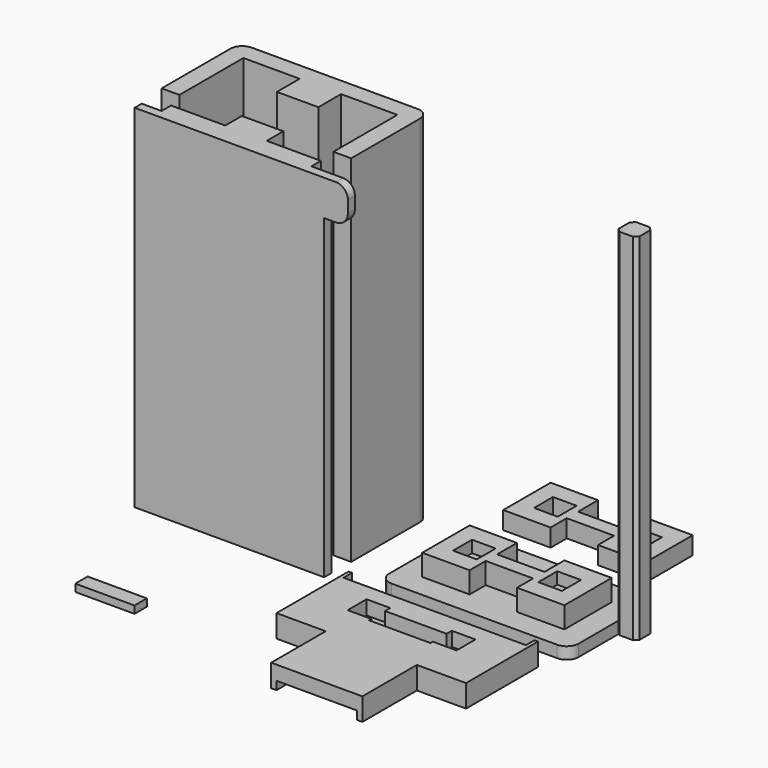
from build123d import *

# Parameters (mm, degrees)
F0_W      = 30.48
F0_H      = 12.7
F1_DEPTH  = 4.572
F2_W      = 5.08
F2_H      = 5.08
F3_DEPTH  = 2.54
F2_H_2    = 1.524
F2_H_3    = 3.81
F2_H_4    = 4.318
F4_DEPTH  = 7.62
F6_DEPTH  = 2.54
F8_DEPTH  = 76.2
F9_W      = 5.08
F9_H      = 5.08
F10_DEPTH = 3.81
F11_W     = 8.89
F11_H     = 6.096
F12_DEPTH = 76.2
F14_DEPTH = 4.826
F15_DEPTH = 1.778
F16_W     = 17.272
F16_H     = 1.778
F17_DEPTH = 3.81
F18_W     = 12.7
F18_H     = 3.302
F19_DEPTH = 1.5875
F20_W     = 8.89
F20_H     = 4.445
F21_DEPTH = 75.438
F22_W     = 1.905
F22_H     = 7.62
F23_DEPTH = 5.08
F24_R     = 2.54
F25_R     = 2.54


# Not quite as in the source:
# - a feature names something its author has since deleted; it is built from what else it names


with BuildPart() as f1:
    # F0 (on Top) → F1 (new body)
    with BuildSketch(Plane.XY):
        Rectangle(F0_W, F0_H)
    extrude(amount=F1_DEPTH)

    # F2 (on face) → F3 (cut)
    with BuildSketch(Plane.XY.offset(4.572)):
        with Locations((-9.144, 0)):
            Rectangle(F2_W, F2_H)
        with Locations((9.144, 0)):
            Rectangle(F2_W, F2_H)
    extrude(amount=-F3_DEPTH, mode=Mode.SUBTRACT)

    # F2 (on face) → F4 (cut)
    with BuildSketch(Plane.XY.offset(4.572)):
        with Locations((-2.54, 1.778)):
            Rectangle(F2_W, F2_H_2)
        with Locations((-2.54, 4.445)):
            Rectangle(F2_W, F2_H_3)
        Polygon((5.08, 6.35), (0, 6.35), (0, 2.54), (0, 1.016), (5.08, 1.016), align=None)
        with Locations((2.54, -4.191)):
            Rectangle(F2_W, F2_H_4)
        with Locations((-2.54, -4.191)):
            Rectangle(F2_W, F2_H_4)
    extrude(amount=-F4_DEPTH, mode=Mode.SUBTRACT)

    # F5 (on face) → F6 (join)
    with BuildSketch(Plane(origin=(0, 0, 0), x_dir=(1, 0, 0), z_dir=(0, 0, -1))):
        with BuildLine():
            Line((-20.32, -6.8208193406), (-20.32, -8.89))
            ThreePointArc((-20.32, -8.89), (-19.5760512242, -10.6860512242), (-17.78, -11.43))
            Line((-17.78, -11.43), (-17.2756779939, -11.43))
            Line((-17.2756779939, -11.43), (17.78, -11.43))
            ThreePointArc((17.78, -11.43), (19.5760512242, -10.6860512242), (20.32, -8.89))
            Line((20.32, -8.89), (20.32, 0))
            Line((20.32, 0), (20.32, 8.89))
            ThreePointArc((20.32, 8.89), (19.5760512242, 10.6860512242), (17.78, 11.43))
            Line((17.78, 11.43), (0, 11.43))
            Line((0, 11.43), (-17.78, 11.43))
            ThreePointArc((-17.78, 11.43), (-19.5760512242, 10.6860512242), (-20.32, 8.89))
            Line((-20.32, 8.89), (-20.32, -6.8208193406))
        make_face()
        Polygon((5.08, 6.35), (15.24, 6.35), (15.24, -6.35), (5.08, -6.35), (5.08, -1.016), (-5.08, -1.016), (-5.08, -6.35), (-15.24, -6.35), (-15.24, 6.35), (-5.08, 6.35), (-5.08, 2.032), (5.08, 2.032), align=None, mode=Mode.SUBTRACT)
        Polygon((15.24, -6.35), (15.24, 6.35), (5.08, 6.35), (5.08, 2.032), (-5.08, 2.032), (-5.08, 6.35), (-15.24, 6.35), (-15.24, -6.35), (-5.08, -6.35), (-5.08, -1.016), (5.08, -1.016), (5.08, -6.35), align=None)
    extrude(amount=F6_DEPTH)


with BuildPart() as f8:
    # F7 (on Top) → F8 (new body)
    with BuildSketch(Plane.XY):
        Polygon((27.4387739635, 1.4605), (26.6767739635, 2.2225), (23.7557739635, 2.2225), (22.9937739635, 1.4605), (22.9937739635, -1.4605), (23.7557739635, -2.2225), (25.2162739635, -2.2225), (26.6767739635, -2.2225), (27.4387739635, -1.4605), (27.4387739635, 0), align=None)
    extrude(amount=F8_DEPTH)


with BuildPart() as f10:
    # F9 (on Top) → F10 (new body)
    with BuildSketch(Plane.XY):
        Polygon((15.24, 15.3667641968), (15.24, 28.0667641968), (5.08, 28.0667641968), (5.08, 22.7327641968), (0, 22.7327641968), (-5.08, 22.7327641968), (-5.08, 24.2567641968), (-5.08, 28.0667641968), (-15.24, 28.0667641968), (-15.24, 15.3667641968), (-5.08, 15.3667641968), (-5.08, 19.6847641968), (0, 19.6847641968), (5.08, 19.6847641968), (5.08, 15.3667641968), align=None)
        with Locations((-9.144, 21.7167641968)):
            Rectangle(F9_W, F9_H, mode=Mode.SUBTRACT)
        with Locations((9.144, 21.7167641968)):
            Rectangle(F9_W, F9_H, mode=Mode.SUBTRACT)
    extrude(amount=F10_DEPTH)


with BuildPart() as f12:
    # F11 (on Top) → F12 (new body)
    with BuildSketch(Plane.XY):
        with Locations((-48.2656806707, 4.572)):
            Rectangle(F11_W, F11_H)
        with BuildLine():
            Line((-43.8206806707, 7.62), (-31.7556806707, 7.62))
            Line((-31.7556806707, 7.62), (-31.7556806707, -7.62))
            Line((-31.7556806707, -7.62), (-31.7556806707, -9.525))
            Line((-31.7556806707, -9.525), (-27.9456806707, -9.525))
            Line((-27.9456806707, -9.525), (-27.9456806707, 8.89))
            ThreePointArc((-27.9456806707, 8.89), (-28.6896294465, 10.6860512242), (-30.4856806707, 11.43))
            Line((-30.4856806707, 11.43), (-66.0456806707, 11.43))
            ThreePointArc((-66.0456806707, 11.43), (-67.841731895, 10.6860512242), (-68.5856806707, 8.89))
            Line((-68.5856806707, 8.89), (-68.5856806707, -9.525))
            Line((-68.5856806707, -9.525), (-64.7756806707, -9.525))
            Line((-64.7756806707, -9.525), (-64.7756806707, -7.62))
            Line((-64.7756806707, -7.62), (-64.7756806707, 7.62))
            Line((-64.7756806707, 7.62), (-52.7106806707, 7.62))
            Line((-52.7106806707, 7.62), (-43.8206806707, 7.62))
        make_face()
    extrude(amount=F12_DEPTH)


with BuildPart() as f14:
    # F13 (on Top) → F14 (new body)
    with BuildSketch(Plane.XY):
        Polygon((9.779, -53.6695963979), (9.779, -39.0645963979), (0, -39.0645963979), (-9.779, -39.0645963979), (-9.779, -53.6695963979), align=None)
        Polygon((-19.558, -22.0465963979), (-19.558, -19.7605963979), (-20.32, -19.7605963979), (-20.32, -39.0645963979), (-9.779, -39.0645963979), (0, -39.0645963979), (0, -31.4445963979), (-6.604, -31.4445963979), (-6.604, -30.8095963979), (-11.684, -30.8095963979), (-11.684, -25.7295963979), (-6.604, -25.7295963979), (-6.604, -27.1265963979), (0, -27.1265963979), (0, -22.0465963979), align=None)
        Polygon((20.32, -39.0645963979), (20.32, -19.7605963979), (19.558, -19.7605963979), (19.558, -22.0465963979), (0, -22.0465963979), (0, -27.1265963979), (6.604, -27.1265963979), (6.604, -25.7295963979), (11.684, -25.7295963979), (11.684, -30.8095963979), (6.604, -30.8095963979), (6.604, -31.4445963979), (0, -31.4445963979), (0, -39.0645963979), (9.779, -39.0645963979), align=None)
    extrude(amount=F14_DEPTH)

    # F13 (on Top) → F15 (join)
    with BuildSketch(Plane.XY):
        Polygon((-6.604, -28.2695963979), (-6.604, -27.1265963979), (-6.604, -25.7295963979), (-11.684, -25.7295963979), (-11.684, -30.8095963979), (-6.604, -30.8095963979), align=None)
        Polygon((6.604, -25.7295963979), (6.604, -27.1265963979), (6.604, -30.8095963979), (11.684, -30.8095963979), (11.684, -25.7295963979), align=None)
    extrude(amount=F15_DEPTH)

    # F16 (on face) → F17 (cut)
    with BuildSketch(Plane.XZ.offset(53.6695963979)):
        with Locations((0, 0.889)):
            Rectangle(F16_W, F16_H)
    extrude(amount=-F17_DEPTH, mode=Mode.SUBTRACT)


with BuildPart() as f19:
    # F18 (on Top) → F19 (new body)
    with BuildSketch(Plane.XY):
        with Locations((-50.8568691254, -45.2617781689)):
            Rectangle(F18_W, F18_H)
    extrude(amount=F19_DEPTH)


with BuildPart() as f21:
    # F20 (on Top) → F21 (new body)
    with BuildSketch(Plane.XY):
        with Locations((-48.3141668069, -10.0349279085)):
            Rectangle(F20_W, F20_H)
        Polygon((-64.3796668069, -14.7974279085), (-32.2486668069, -14.7974279085), (-32.2486668069, -12.2574279085), (-43.8691668069, -12.2574279085), (-52.7591668069, -12.2574279085), (-64.3796668069, -12.2574279085), align=None)
        Polygon((-68.6341668069, -16.7024279085), (-27.9941668069, -16.7024279085), (-27.9941668069, -14.7974279085), (-32.2486668069, -14.7974279085), (-64.3796668069, -14.7974279085), (-68.6341668069, -14.7974279085), align=None)
    extrude(amount=F21_DEPTH)

    # F22 (on face) → F23 (join)
    with BuildSketch(Plane.YZ.offset(-27.9941668069)):
        with Locations((-15.7499279085, 71.628)):
            Rectangle(F22_W, F22_H)
    extrude(amount=F23_DEPTH)

    # F24
    f24_edges = [f21.edges().sort_by_distance(p)[0] for p in [
        (-22.914167, -15.749928, 75.438),
    ]]
    fillet(f24_edges, radius=F24_R)

    # F25
    f25_edges = [f21.edges().sort_by_distance(p)[0] for p in [
        (-22.914167, -15.749928, 67.818),
    ]]
    fillet(f25_edges, radius=F25_R)


solid = Compound([f1.part, f8.part, f10.part, f12.part, f14.part, f19.part, f21.part])
